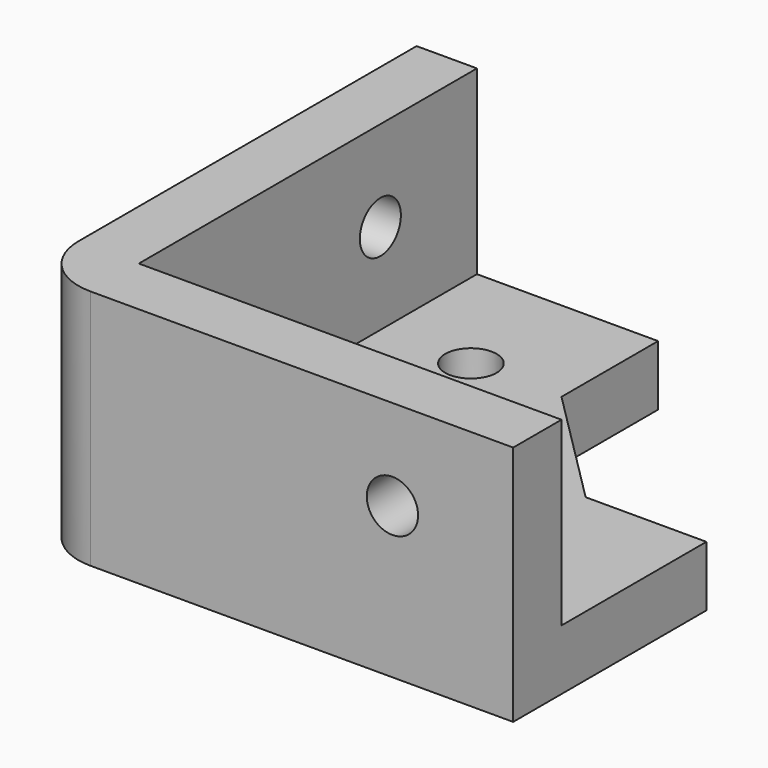
from build123d import *

# Parameters (mm, degrees)
F0_R     = 2.125
F1_DEPTH = 5
F3_DEPTH = 15
F4_SIZE  = 10
F5_R     = 2.125
F6_DEPTH = 5
F7_R     = 2.125
F8_DEPTH = 5
F9_R     = 5


with BuildPart() as f1:
    # F0 (on Top) → F1 (new body)
    with BuildSketch(Plane.XY):
        Polygon((0, 20), (0, 40), (-20, 40), (-20, 0), (20, 0), (20, 20), align=None)
        with Locations((10, 12.5)):
            Circle(F0_R, mode=Mode.SUBTRACT)
        with Locations((-7.5, 30)):
            Circle(F0_R, mode=Mode.SUBTRACT)
    extrude(amount=F1_DEPTH)

    # F2 (on face) → F3 (join)
    with BuildSketch(Plane.XY.offset(5)):
        Polygon((-15, 40), (-20, 40), (-20, 0), (20, 0), (20, 5), (-15, 5), align=None)
    extrude(amount=F3_DEPTH)

    # F4
    f4_edges = [f1.edges().sort_by_distance(p)[0] for p in [
        (0, 20, 2.5),
    ]]
    chamfer(f4_edges, length=F4_SIZE)

    # F5 (on face) → F6 (cut)
    with BuildSketch(Plane.XZ):
        with Locations((10, 12.5)):
            Circle(F5_R)
    extrude(amount=-F6_DEPTH, mode=Mode.SUBTRACT)

    # F7 (on face) → F8 (cut)
    with BuildSketch(Plane(origin=(-20, 0, 0), x_dir=(0, -1, 0), z_dir=(-1, 0, 0))):
        with Locations((-30, 12.5)):
            Circle(F7_R)
    extrude(amount=-F8_DEPTH, mode=Mode.SUBTRACT)

    # F9
    f9_edges = [f1.edges().sort_by_distance(p)[0] for p in [
        (-20, 0, 10),
    ]]
    fillet(f9_edges, radius=F9_R)


solid = f1.part
